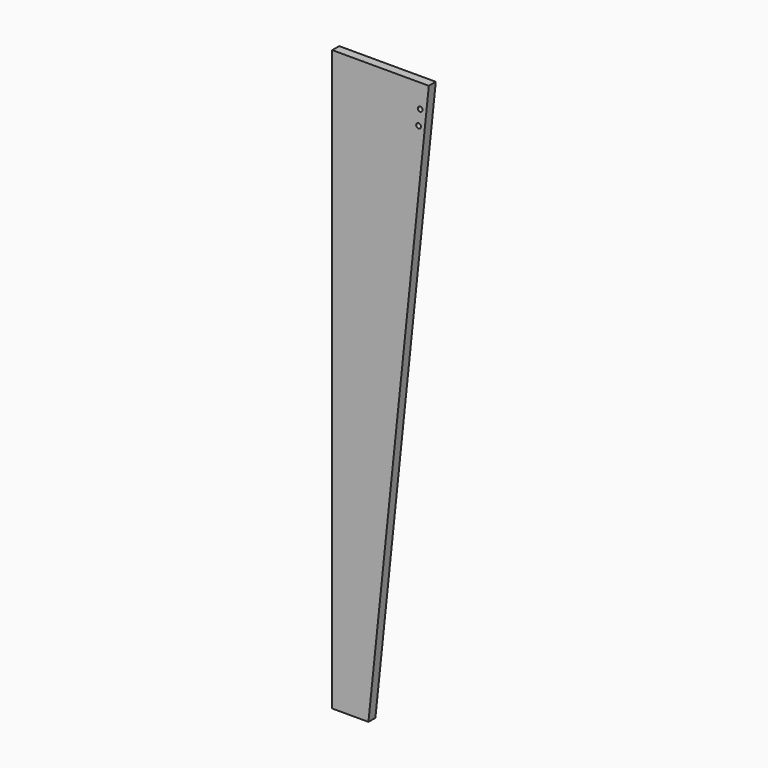
from build123d import *

# Parameters (mm, degrees)
F2_DEPTH = 18.288
F4_D     = 10
F4_DEPTH = 11.5
F4_TIP   = 3.0043030951


# Not quite as in the source:
# - a variable given as a bare number and used for a length is read in inches; the dataset says mm whatever the document's units were


with BuildPart() as f2:
    # F0 (on Front) → F2 (new body)
    with BuildSketch(Plane.XZ):
        Polygon((-304.6112403404, 1131.9026269978), (-304.6112403404, -87.2973730022), (-228.4112403404, -87.2973730022), (-101.4112403404, 1131.9026269978), align=None)
    extrude(amount=F2_DEPTH)

    # F4
    with Locations(Plane.XZ.offset(18.288)):
        with Locations((-119.6044687363, 1082.7228909215), (-122.9198634326, 1050.895101837)):
            Hole(F4_D / 2, depth=F4_DEPTH)
            with Locations((0, 0, -(F4_DEPTH + F4_TIP / 2))):  # 118° drill point
                Cone(0, F4_D / 2, F4_TIP, mode=Mode.SUBTRACT)


solid = f2.part
